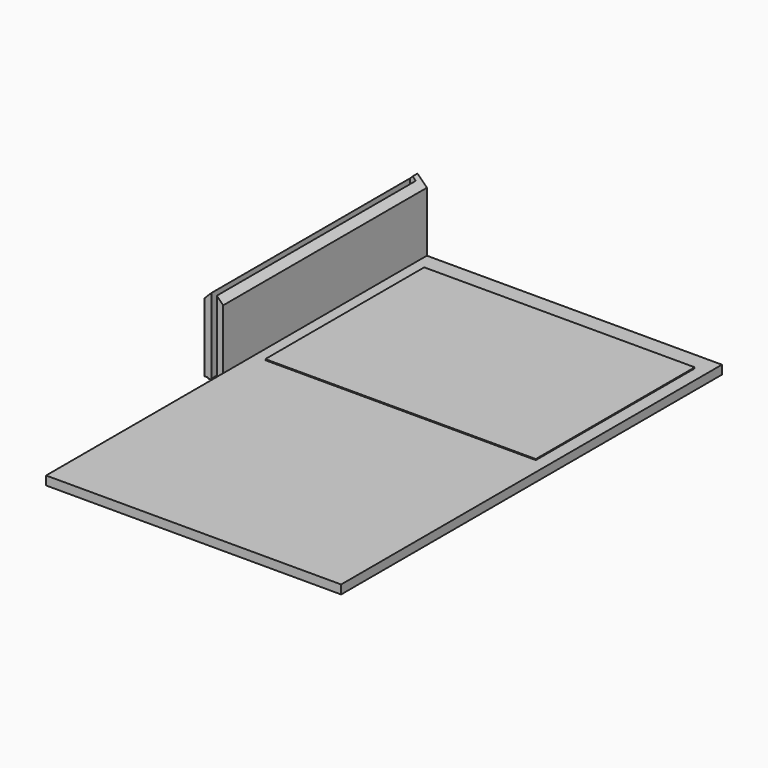
from build123d import *

# Parameters (mm, degrees)
F0_W        = 76.5407979488
F0_H        = 123.4830245376
F1_DEPTH    = 2.286
F3_DEPTH    = 20.32
F4_W        = 70.1841525733
F4_H        = 51.5401670709
F5_DEPTH    = 2.54
F6_W        = 3.1785480678
F6_H        = 64.6996945143
F7_DEPTH    = 0.2286
F8_T1_DEPTH = 79.1161617244


# Not quite as in the source:
# - a fillet or chamfer that OpenCascade refuses, or shapes differently, is made with other operations: its cross-section is extruded or revolved along the edge and cut away or added


with BuildPart() as f1:
    # F0 (on Top) → F1 (new body)
    with BuildSketch(Plane.XY):
        with Locations((1.9688718021, 4.2612589896)):
            Rectangle(F0_W, F0_H)
    extrude(amount=F1_DEPTH)

    # F4 (on Top) → F5 (join)
    with BuildSketch(Plane.XY):
        with Locations((1.8656272441, 35.5202662759)):
            Rectangle(F4_W, F4_H)
    extrude(amount=F5_DEPTH)


with BuildPart() as f3:
    # F2 (on Top) → F3 (new body)
    with BuildSketch(Plane.XY):
        Polygon((-36.3286137581, 0), (-36.3286137581, 66.0520121455), (-41.2212088704, 66.0520121455), (-41.2212088704, 0), (-39.4303016365, 0), (-39.4303016365, 64.5106732845), (-37.9857048392, 64.5106732845), (-37.9857048392, 0), align=None)
    extrude(amount=F3_DEPTH)

    # F6 (on Top) → F7 (join)
    with BuildSketch(Plane.XY):
        with Locations((-38.7550909072, 32.3498472571)):
            Rectangle(F6_W, F6_H)
    extrude(amount=-F7_DEPTH)

    # F8: chamfer of 2.54 on 2 edges, made by hand

    # F8_s2 → F8_t1 (cut)
    with BuildSketch(Plane.XZ.offset(-72.584086935)):
        Polygon((-36.3286137581, 17.78), (-38.8686137581, 20.32), (-36.3286137581, 20.32), align=None)
        Polygon((-38.6812088704, 20.32), (-41.2212088704, 17.78), (-41.2212088704, 20.32), align=None)
    extrude(amount=F8_T1_DEPTH, mode=Mode.SUBTRACT)


solid = Compound([f1.part, f3.part])
